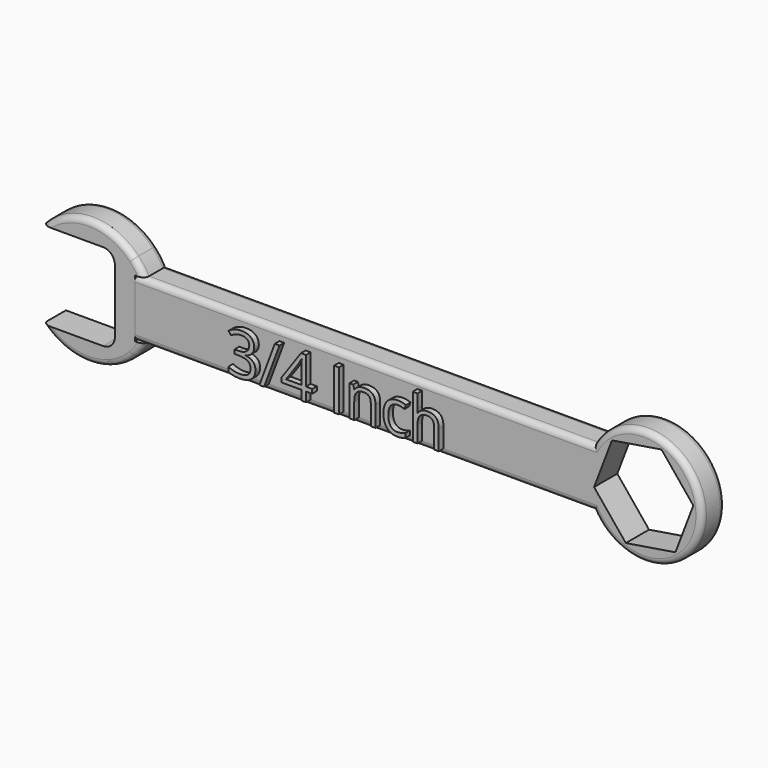
from build123d import *

# Parameters (mm, degrees)
F1_DEPTH     = 6.35
F3_DEPTH     = 6.35
F4_R         = 1.27
F4_2_R       = 1.27
F5_R         = 2.54
F6_TEXT_SIZE = 12.7
F7_DEPTH     = 1.27


# Not quite as in the source:
# - Text() gives the source's letters only with a copy of the font that has no kerning and outlines rounded to 1/6400 em; it was checked with that copy


with BuildPart() as f1:
    # F0 (on Front) → F1 (new body)
    with BuildSketch(Plane.XZ):
        with BuildLine():
            Line((0, 6.35), (-50.1896717561, 6.35))
            Line((-50.1896717561, 6.35), (-50.1896717561, -6.35))
            Line((-50.1896717561, -6.35), (50.1896717561, -6.35))
            ThreePointArc((50.1896717561, -6.35), (73.8881943841, 0), (50.1896717561, 6.35))
            Line((50.1896717561, 6.35), (0, 6.35))
        make_face()
        Polygon((65.0980562836, 10.2801011633), (72.0459540947, 1.7540108514), (68.1360921953, -8.5260903119), (57.2783324847, -10.2801011633), (50.3304346735, -1.7540108514), (54.240296573, 8.5260903119), align=None, mode=Mode.SUBTRACT)
    extrude(amount=F1_DEPTH)

    # F4
    f4_edges = [f1.edges().sort_by_distance(p)[0] for p in [
        (0, -6.35, -6.35),
        (0, -6.35, 6.35),
        (73.888194, -6.35, 0),
        (0, 0, -6.35),
        (0, 0, 6.35),
        (73.888194, 0, 0),
    ]]
    fillet(f4_edges, radius=F4_R)

    # F6 (on face) → F7 (join)
    with BuildSketch(Plane.XZ.offset(6.35)):
        with Locations((-29.293656525, -5.08)):
            Text('3/4 Inch', F6_TEXT_SIZE, font='Open Sans', text_align=(TextAlign.LEFT, TextAlign.BOTTOM))
    extrude(amount=F7_DEPTH)


with BuildPart() as f3:
    # F2 (on face) → F3 (new body)
    with BuildSketch(Plane.XZ.offset(6.35)):
        with BuildLine():
            Line((-54.5556657016, -9.525), (-70.3492404227, -9.525))
            ThreePointArc((-70.3492404227, -9.525), (-60.3496717561, -13.8100325314), (-50.3501030894, -9.525))
            ThreePointArc((-50.3501030894, -9.525), (-49.105486735, -8.01781153), (-48.0861282829, -6.35))
            Line((-48.0861282829, -6.35), (-50.1896717561, -6.35))
            Line((-50.1896717561, -6.35), (-50.1896717561, 6.35))
            Line((-50.1896717561, 6.35), (-48.0861282829, 6.35))
            ThreePointArc((-48.0861282829, 6.35), (-49.105486735, 8.01781153), (-50.3501030894, 9.525))
            ThreePointArc((-50.3501030894, 9.525), (-60.3496717561, 13.8100325314), (-70.3492404227, 9.525))
            Line((-70.3492404227, 9.525), (-54.5556657016, 9.525))
            Line((-54.5556657016, 9.525), (-54.5556657016, -9.525))
        make_face()
    extrude(amount=-F3_DEPTH)

    # F4#2
    f4_2_edges = [f3.edges().sort_by_distance(p)[0] for p in [
        (-58.399915, 0, 13.671702),
        (-58.399915, -6.35, 13.671702),
        (-58.399915, -6.35, -13.671702),
    ]]
    fillet(f4_2_edges, radius=F4_2_R)

    # F5
    f5_edges = [f3.edges().sort_by_distance(p)[0] for p in [
        (-54.555666, -3.175, 9.525),
        (-54.555666, -3.175, -9.525),
    ]]
    fillet(f5_edges, radius=F5_R)


solid = Compound([f1.part, f3.part])
